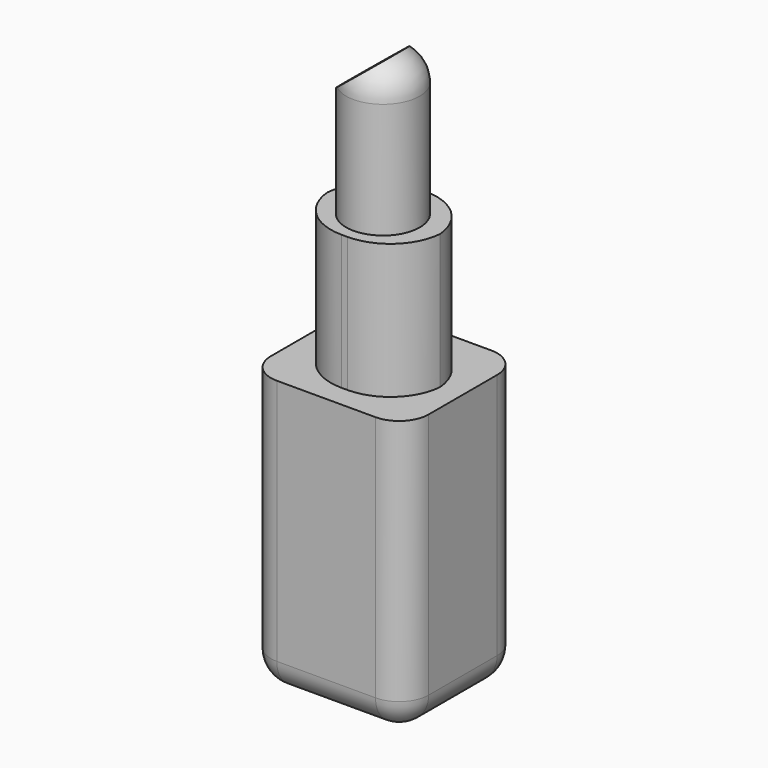
from build123d import *

# Parameters (mm, degrees)
F0_R         = 46.2156340315
F1_DEPTH     = 68.834
F2_R         = 33.7265634664
F4_W         = 27.1566789597
F4_H         = 47.5971903652
F5_DEPTH     = 24.892
F6_R         = 5.08
F7_R         = 5.08
F8_W         = 19.4552922621
F8_H         = 16.8696646579
F9_DEPTH     = 51.816
F10_T1_DEPTH = 97.8067683632
F11_R        = 5.3006376135
F12_DEPTH    = 66.802
F13_SIZE     = 5.08
F14_R        = 6.3300692049
F15_DEPTH    = 25.4
F16_R        = 5.5188922036
F18_DEPTH    = 26.416


# Not quite as in the source:
# - a fillet or chamfer that OpenCascade refuses, or shapes differently, is made with other operations: its cross-section is extruded or revolved along the edge and cut away or added


with BuildPart() as f1:
    # F0 (on Front) → F1 (new body)
    with BuildSketch(Plane.XZ):
        Circle(F0_R)
    extrude(amount=F1_DEPTH)

    # F2
    f2_edges = [f1.edges().sort_by_distance(p)[0] for p in [
        (46.215634, -34.417, 0),
        (-46.215634, 0, 0),
        (-46.215634, -68.834, 0),
    ]]
    fillet(f2_edges, radius=F2_R)


with BuildPart() as f5:
    # F4 (on Front) → F5 (new body)
    with BuildSketch(Plane.XZ):
        with Locations((-0.1460043713, 4.81812004)):
            Rectangle(F4_W, F4_H)
    extrude(amount=F5_DEPTH)

    # F6
    f6_edges = [f5.edges().sort_by_distance(p)[0] for p in [
        (13.432335, -24.892, 4.81812),
        (13.432335, 0, 4.81812),
        (-13.724344, 0, 4.81812),
        (-13.724344, -24.892, 4.81812),
    ]]
    fillet(f6_edges, radius=F6_R)

    # F7
    f7_edges = [f5.edges().sort_by_distance(p)[0] for p in [
        (-12.236446, -23.404102, -18.980475),
    ]]
    fillet(f7_edges, radius=F7_R)


with BuildPart() as f9:
    # F8 (on Top) → F9 (new body)
    with BuildSketch(Plane.XY):
        with Locations((-0.0383681618, -12.6372461673)):
            Rectangle(F8_W, F8_H)
    extrude(amount=F9_DEPTH)

    # F10: fillet of radius 9.1981536726 on 4 edges, made by hand

    # F10_s2 → F10_t1 (cut)
    with BuildSketch(Plane.XY.offset(-22.9953841816)):
        with BuildLine():
            ThreePointArc((9.6892779693, -13.400567511), (6.995201133, -6.8964906747), (0.4911242967, -4.2024138384))
            Line((0.4911242967, -4.2024138384), (9.6892779693, -4.2024138384))
            Line((9.6892779693, -4.2024138384), (9.6892779693, -13.400567511))
        make_face()
        with BuildLine():
            ThreePointArc((9.6892779693, -11.8739248236), (6.995201133, -18.3780016599), (0.4911242967, -21.0720784962))
            Line((0.4911242967, -21.0720784962), (9.6892779693, -21.0720784962))
            Line((9.6892779693, -21.0720784962), (9.6892779693, -11.8739248236))
        make_face()
        with BuildLine():
            ThreePointArc((-0.5678606202, -4.2024138384), (-7.0719374565, -6.8964906747), (-9.7660142928, -13.400567511))
            Line((-9.7660142928, -13.400567511), (-9.7660142928, -4.2024138384))
            Line((-9.7660142928, -4.2024138384), (-0.5678606202, -4.2024138384))
        make_face()
        with BuildLine():
            ThreePointArc((-9.7660142928, -11.8739248236), (-7.0719374565, -18.3780016599), (-0.5678606202, -21.0720784962))
            Line((-0.5678606202, -21.0720784962), (-9.7660142928, -21.0720784962))
            Line((-9.7660142928, -21.0720784962), (-9.7660142928, -11.8739248236))
        make_face()
    extrude(amount=F10_T1_DEPTH, mode=Mode.SUBTRACT)


with BuildPart() as f12:
    # F11 (on Top) → F12 (new body)
    with BuildSketch(Plane.XY):
        with Locations((0, -13.1403291598)):
            Circle(F11_R)
    extrude(amount=F12_DEPTH)

    # F13
    f13_edges = [f12.edges().sort_by_distance(p)[0] for p in [
        (-5.300638, -13.140329, 66.802),
    ]]
    chamfer(f13_edges, length=F13_SIZE)


with BuildPart() as f15:
    # F14 (on face) → F15 (new body)
    with BuildSketch(Plane.XY.offset(51.816)):
        with Locations((0, -12.8519842401)):
            Circle(F14_R)
    extrude(amount=F15_DEPTH)

    # F16
    f16_edges = [f15.edges().sort_by_distance(p)[0] for p in [
        (-6.330069, -12.851984, 77.216),
    ]]
    fillet(f16_edges, radius=F16_R)

    # F17 (on Front) → F18 (cut)
    with BuildSketch(Plane.XZ):
        Polygon((-14.298915863, 84.5396593213), (-9.31422133, 67.3583671451), (7.7610081062, 81.2518820167), align=None)
    extrude(amount=F18_DEPTH, mode=Mode.SUBTRACT)


solid = Compound([f5.part, f9.part, f12.part, f15.part])
